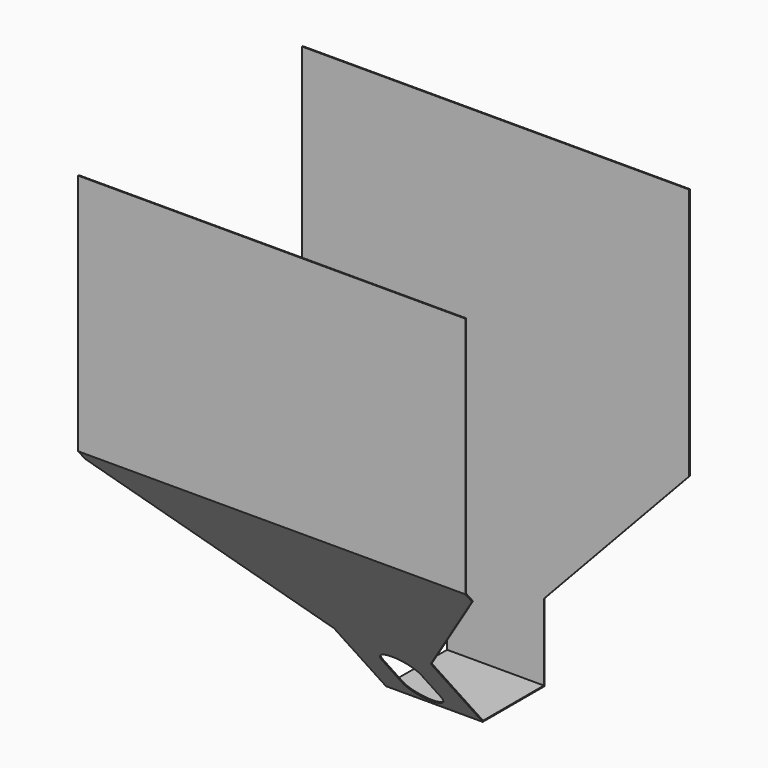
from build123d import *

# Parameters (mm, degrees)
F1_DEPTH = 400
F3_DEPTH = 290.001
F5_DEPTH = 161.870333055


# Not quite as in the source:
# - a feature names something its author has since deleted; it is built from what else it names


with BuildPart() as f1:
    # F0 (on Right) → F1 (new body)
    with BuildSketch(Plane.YZ):
        Polygon((-80, 0), (0, 0), (0, 501), (-1, 501), (-1, 1), (-79.5336923418, 1), (-289, 250.6322246791), (-289, 501), (-290, 501), (-290, 250.2682544448), align=None)
    extrude(amount=-F1_DEPTH)

    # F2 (on face) → F3 (cut, through all)
    with BuildSketch(Plane(origin=(0, 0, 0), x_dir=(-1, 0, 0), z_dir=(0, 1, 0))):
        Polygon((400, 0), (400, 240), (250, 80), (250, 0), align=None)
        Polygon((0, 0), (150, 0), (150, 80), (0, 240), align=None)
    extrude(amount=-F3_DEPTH, mode=Mode.SUBTRACT)

    # F4 (on face) → F5 (cut, through all)
    with BuildSketch(Plane(origin=(0, -46.1798826636, -38.7495225108), x_dir=(-1, 0, 0), z_dir=(0, 0.7660444431, 0.6427876097))):
        with BuildLine():
            Line((180, 116.8893164331), (180, 76.8893164331))
            ThreePointArc((180, 76.8893164331), (200, 56.8893164331), (220, 76.8893164331))
            Line((220, 76.8893164331), (220, 116.8893164331))
            ThreePointArc((220, 116.8893164331), (200, 136.8893164331), (180, 116.8893164331))
        make_face()
    extrude(amount=-F5_DEPTH, mode=Mode.SUBTRACT)


solid = f1.part
